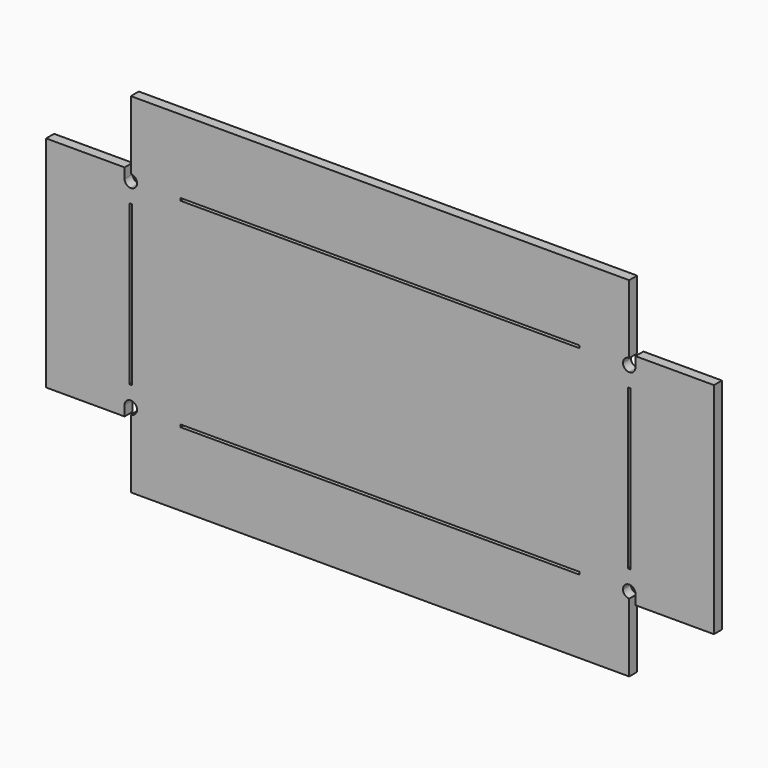
from build123d import *

# Parameters (mm, degrees)
F1_W     = 20.0025
F1_H     = 2.54
F2_DEPTH = 2.54


# Not quite as in the source:
# - a variable given as a bare number and used for a length is read in inches; the dataset says mm whatever the document's units were


with BuildPart() as f2:
    # F1 (on Front) → F2 (new body)
    with BuildSketch(Plane.XZ):
        with Locations((-11.58875, -1.27)):
            Rectangle(F1_W, F1_H)
        with Locations((-11.58875, 52.07)):
            Rectangle(F1_W, F1_H)
        with Locations((138.58875, 52.07)):
            Rectangle(F1_W, F1_H)
        with Locations((138.58875, -1.27)):
            Rectangle(F1_W, F1_H)
        with BuildLine():
            ThreePointArc((-1.5875, 0), (-1.1225320151, 1.1225320151), (0, 1.5875))
            Line((0, 1.5875), (0, 5.08))
            Line((0, 5.08), (-0.3175, 5.08))
            Line((-0.3175, 5.08), (-0.3175, 45.72))
            Line((-0.3175, 45.72), (0, 45.72))
            Line((0, 45.72), (0, 49.2125))
            ThreePointArc((0, 49.2125), (-1.1225320151, 49.6774679849), (-1.5875, 50.8))
            Line((-1.5875, 50.8), (-21.59, 50.8))
            Line((-21.59, 50.8), (-21.59, 0))
            Line((-21.59, 0), (-1.5875, 0))
        make_face()
        with BuildLine():
            Line((127, 5.08), (127, 1.5875))
            ThreePointArc((127, 1.5875), (128.1225320151, 1.1225320151), (128.5875, 0))
            Line((128.5875, 0), (148.59, 0))
            Line((148.59, 0), (148.59, 50.8))
            Line((148.59, 50.8), (128.5875, 50.8))
            ThreePointArc((128.5875, 50.8), (128.1225320151, 49.6774679849), (127, 49.2125))
            Line((127, 49.2125), (127, 45.72))
            Line((127, 45.72), (127.3175, 45.72))
            Line((127.3175, 45.72), (127.3175, 5.08))
            Line((127.3175, 5.08), (127, 5.08))
        make_face()
        with BuildLine():
            Line((12.7, 0), (1.5875, 0))
            ThreePointArc((1.5875, 0), (1.1225320151, -1.1225320151), (0, -1.5875))
            Line((0, -1.5875), (0, -2.54))
            Line((0, -2.54), (0, -19.05))
            Line((0, -19.05), (127, -19.05))
            Line((127, -19.05), (127, -2.54))
            Line((127, -2.54), (127, -1.5875))
            ThreePointArc((127, -1.5875), (125.8774679849, -1.1225320151), (125.4125, 0))
            Line((125.4125, 0), (114.3, 0))
            Line((114.3, 0), (114.3, -0.3175))
            Line((114.3, -0.3175), (12.7, -0.3175))
            Line((12.7, -0.3175), (12.7, 0))
        make_face()
        with BuildLine():
            ThreePointArc((0, 52.3875), (1.1225320151, 51.9225320151), (1.5875, 50.8))
            Line((1.5875, 50.8), (12.7, 50.8))
            Line((12.7, 50.8), (12.7, 51.1175))
            Line((12.7, 51.1175), (114.3, 51.1175))
            Line((114.3, 51.1175), (114.3, 50.8))
            Line((114.3, 50.8), (125.4125, 50.8))
            ThreePointArc((125.4125, 50.8), (125.8774679849, 51.9225320151), (127, 52.3875))
            Line((127, 52.3875), (127, 53.34))
            Line((127, 53.34), (127, 69.85))
            Line((127, 69.85), (0, 69.85))
            Line((0, 69.85), (0, 53.34))
            Line((0, 53.34), (0, 52.3875))
        make_face()
        with BuildLine():
            ThreePointArc((0, 1.5875), (1.1225320151, 1.1225320151), (1.5875, 0))
            Line((1.5875, 0), (12.7, 0))
            Line((12.7, 0), (12.7, 0.3175))
            Line((12.7, 0.3175), (114.3, 0.3175))
            Line((114.3, 0.3175), (114.3, 0))
            Line((114.3, 0), (125.4125, 0))
            ThreePointArc((125.4125, 0), (125.8774679849, 1.1225320151), (127, 1.5875))
            Line((127, 1.5875), (127, 5.08))
            Line((127, 5.08), (126.6825, 5.08))
            Line((126.6825, 5.08), (126.6825, 45.72))
            Line((126.6825, 45.72), (127, 45.72))
            Line((127, 45.72), (127, 49.2125))
            ThreePointArc((127, 49.2125), (125.8774679849, 49.6774679849), (125.4125, 50.8))
            Line((125.4125, 50.8), (114.3, 50.8))
            Line((114.3, 50.8), (114.3, 50.4825))
            Line((114.3, 50.4825), (12.7, 50.4825))
            Line((12.7, 50.4825), (12.7, 50.8))
            Line((12.7, 50.8), (1.5875, 50.8))
            ThreePointArc((1.5875, 50.8), (1.1225320151, 49.6774679849), (0, 49.2125))
            Line((0, 49.2125), (0, 45.72))
            Line((0, 45.72), (0.3175, 45.72))
            Line((0.3175, 45.72), (0.3175, 5.08))
            Line((0.3175, 5.08), (0, 5.08))
            Line((0, 5.08), (0, 1.5875))
        make_face()
    extrude(amount=F2_DEPTH)


solid = f2.part
